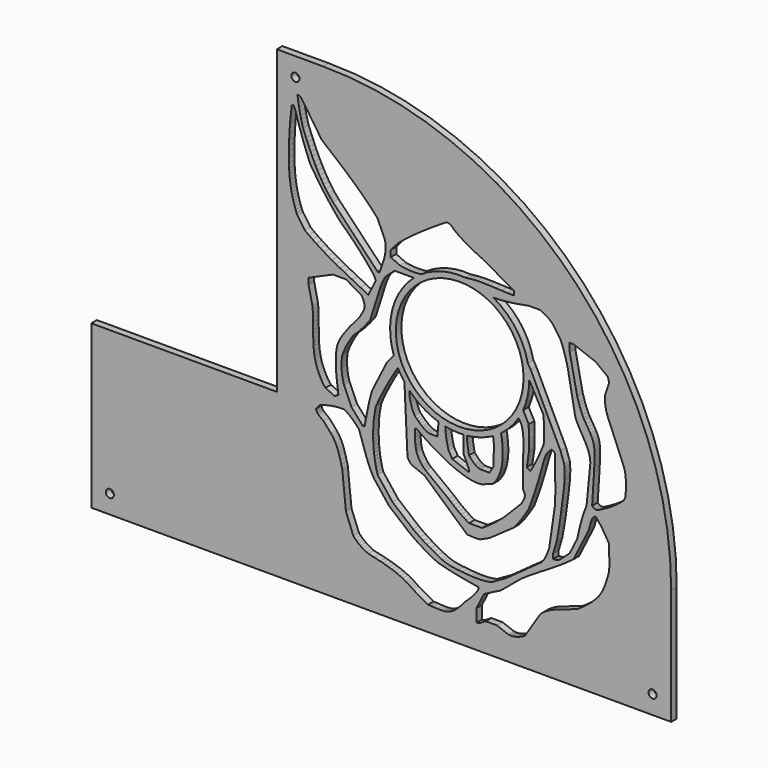
from build123d import *

# Parameters (mm, degrees)
F0_R     = 1.75
F0_R_2   = 27.531271
F1_DEPTH = 3


# Not quite as in the source:
# - ends of sketch curves that miss each other by under 0.0002 mm in the source are joined


with BuildPart() as f1:
    # F0 (on Front) → F1 (new body)
    with BuildSketch(Plane.XZ):
        with BuildLine():
            Line((-25, 100), (-45, 100))
            Line((-45, 100), (-45, -30))
            Line((-45, -30), (-125, -30))
            Line((-125, -30), (-125, -100))
            Line((-125, -100), (125, -100))
            Line((125, -100), (125, -50))
            ThreePointArc((125, -50), (81.066017178, 56.066017178), (-25, 100))
        make_face()
        with Locations((-117, -92)):
            Circle(F0_R, mode=Mode.SUBTRACT)
        Polygon((-31.287949, 17.776814), (-20.835395, 22.366186), (-15.207096, 22.366186), (-8.774755, 18.694689), (-8.557255, 18.433574), (-8.358189, 18.168406), (-8.176948, 17.89932), (-8.012925, 17.626449), (-7.865514, 17.349925), (-7.734107, 17.069883), (-7.618096, 16.786456), (-7.516876, 16.499777), (-7.356374, 15.9172), (-7.247744, 15.323219), (-7.186129, 14.718902), (-7.16667, 14.105317), (-7.502032, 13.354527), (-7.849095, 12.614687), (-8.211531, 11.889235), (-8.593012, 11.181607), (-8.997212, 10.495239), (-9.427801, 9.833569), (-9.888453, 9.200034), (-10.38284, 8.59807), (-13.599011, 4.926573), (-14.451265, 3.745074), (-15.324612, 2.564526), (-16.187258, 1.372942), (-16.604634, 0.769266), (-17.007414, 0.158336), (-17.391623, -0.461346), (-17.753288, -1.091279), (-18.088435, -1.732961), (-18.39309, -2.38789), (-18.663278, -3.057565), (-18.895027, -3.743484), (-19.084362, -4.447144), (-19.227309, -5.170046), (-19.379026, -6.24827), (-19.488623, -7.330374), (-19.559357, -8.415861), (-19.594481, -9.504236), (-19.597251, -10.595003), (-19.570922, -11.687668), (-19.518749, -12.781734), (-19.443987, -13.876707), (-19.34989, -14.97209), (-19.239714, -16.067389), (-18.984143, -18.255751), (-18.423267, -22.609659), (-20.031352, -23.527533), (-24.051565, -21.691785), (-24.559491, -21.073539), (-25.027916, -20.429124), (-25.461461, -19.761602), (-25.864748, -19.074035), (-26.242397, -18.369483), (-26.599031, -17.651009), (-26.93927, -16.921673), (-27.267736, -16.184538), (-27.549789, -15.504402), (-27.80476, -14.816116), (-28.034023, -14.120071), (-28.238954, -13.416661), (-28.420928, -12.706275), (-28.581319, -11.989306), (-28.721501, -11.266144), (-28.842851, -10.537182), (-28.946742, -9.802812), (-29.03455, -9.063423), (-29.167415, -7.571159), (-29.252444, -6.063523), (-29.300635, -4.543646), (-29.322988, -3.014661), (-29.330501, -1.479699), (-29.345002, 1.595628), (-29.373987, 3.129728), (-29.432126, 4.657278), (-29.530419, 6.175144), (-29.679864, 7.680196), (-31.287949, 15.023191), align=None, mode=Mode.SUBTRACT)
        Polygon((-17.33139, -27.224259), (-16.011139, -27.199031), (-15.552943, -27.469295), (-15.103782, -27.751451), (-14.231239, -28.349693), (-13.390862, -28.990273), (-12.580003, -29.669707), (-11.796014, -30.384509), (-11.036249, -31.131194), (-10.298059, -31.906279), (-9.578798, -32.706277), (-8.856422, -34.825598), (-8.152829, -36.957361), (-7.44696, -39.087617), (-6.717758, -41.202414), (-6.337826, -42.249657), (-5.944164, -43.287804), (-5.53414, -44.315111), (-5.105121, -45.329834), (-4.654476, -46.33023), (-4.179572, -47.314555), (-3.677776, -48.281065), (-3.146457, -49.228017), (3.285885, -57.488886), (12.130354, -64.831881), (13.575378, -65.896058), (15.042077, -66.909543), (16.528551, -67.876781), (18.032897, -68.802218), (19.553215, -69.6903), (21.087605, -70.545473), (22.634164, -71.372184), (24.190993, -72.174876), (26.382616, -72.770954), (28.581654, -73.31486), (30.787186, -73.813088), (32.998288, -74.272132), (35.214037, -74.698489), (37.433509, -75.098651), (39.655782, -75.479115), (41.879931, -75.846374), (41.879931, -76.764248), (41.589377, -77.243893), (41.287323, -77.708872), (40.974487, -78.160098), (40.651581, -78.598481), (39.978425, -79.440371), (39.273575, -80.241836), (38.542751, -81.010173), (37.791672, -81.752678), (37.02606, -82.476644), (36.251633, -83.189369), (35.355307, -84.217706), (34.44471, -85.245054), (33.511446, -86.239737), (33.033689, -86.714929), (32.547117, -87.170077), (32.050679, -87.60122), (31.543326, -88.004399), (31.024008, -88.375654), (30.491675, -88.711026), (29.945278, -89.006555), (29.383768, -89.258282), (28.806094, -89.462247), (28.211206, -89.61449), (27.715774, -89.704496), (27.218513, -89.771301), (26.719612, -89.817304), (26.219261, -89.844906), (25.214965, -89.854507), (24.207137, -89.819304), (22.18694, -89.691295), (21.177599, -89.636892), (20.17078, -89.61449), (13.738439, -85.942992), (13.194491, -85.539999), (12.644397, -85.153792), (12.088389, -84.783813), (11.526702, -84.429503), (10.959569, -84.090301), (10.387223, -83.76565), (9.227827, -83.15776), (8.050382, -82.601361), (6.856755, -82.09198), (5.648815, -81.625142), (4.428429, -81.196375), (3.197465, -80.801206), (1.95779, -80.435161), (0.711273, -80.093766), (-0.54022, -79.77255), (-3.050659, -79.172757), (-5.558584, -78.599997), (-6.457527, -78.203947), (-7.335221, -77.75418), (-8.188733, -77.252179), (-9.015132, -76.699429), (-9.811483, -76.097415), (-10.574854, -75.44762), (-11.302313, -74.751528), (-11.990926, -74.010625), (-15.207096, -65.749756), (-16.815181, -50.145891), (-17.222247, -48.5181), (-17.644987, -46.891312), (-18.103559, -45.284488), (-18.352581, -44.494488), (-18.618121, -43.716591), (-18.902698, -42.953166), (-19.208831, -42.206583), (-19.539042, -41.479214), (-19.895849, -40.773428), (-20.281772, -40.091596), (-20.699331, -39.436087), (-21.151046, -38.809273), (-21.639437, -38.213524), (-24.855608, -34.542026), (-25.389784, -34.150193), (-25.939985, -33.756238), (-26.479319, -33.351638), (-26.980894, -32.927865), (-27.209118, -32.706124), (-27.417819, -32.476393), (-27.603634, -32.237606), (-27.763202, -31.988697), (-27.893162, -31.728601), (-27.990152, -31.456251), (-28.050812, -31.170582), (-28.071778, -30.870529), (-26.463693, -29.03478), (-25.818544, -28.7986), (-25.172194, -28.58034), (-24.524669, -28.379631), (-23.875993, -28.196101), (-23.226191, -28.029381), (-22.575288, -27.879101), (-21.923308, -27.74489), (-21.270276, -27.626378), (-20.616218, -27.523195), (-19.961157, -27.434971), (-18.648129, -27.301919), align=None, mode=Mode.SUBTRACT)
        with Locations((117, -92)):
            Circle(F0_R, mode=Mode.SUBTRACT)
        Polygon((92.357364, -32.717578), (92.534618, -32.706277), (93.335017, -33.659188), (94.098567, -34.642419), (94.829855, -35.652194), (95.533468, -36.68474), (96.213994, -37.736283), (96.876019, -38.803048), (98.162916, -40.967147), (98.180748, -42.345341), (98.224052, -43.725509), (98.325946, -46.48703), (98.353967, -47.866014), (98.346325, -49.242233), (98.324354, -49.928936), (98.287736, -50.614503), (98.23456, -51.298787), (98.162916, -51.98164), (97.725667, -53.479835), (97.274925, -54.976121), (96.793754, -56.454111), (96.536465, -57.181125), (96.265217, -57.897421), (95.977893, -58.600949), (95.672376, -59.289663), (95.346548, -59.961513), (94.998294, -60.614453), (94.625495, -61.246432), (94.226035, -61.855404), (93.797795, -62.439321), (93.33866, -62.996133), (92.840296, -63.551141), (92.332649, -64.089762), (91.816155, -64.612763), (91.291249, -65.12091), (90.758363, -65.61497), (90.217932, -66.095709), (89.116173, -67.020293), (87.989446, -67.900793), (86.841224, -68.743344), (85.674982, -69.554078), (84.494191, -70.339128), (74.041637, -74.010625), (73.269796, -74.367475), (72.506218, -74.736675), (71.75653, -75.126636), (71.026358, -75.545764), (70.321327, -76.002469), (69.979997, -76.24754), (69.647063, -76.505158), (69.323227, -76.776374), (69.009192, -77.06224), (68.705661, -77.363806), (68.413339, -77.682123), (61.980997, -87.778741), (61.097449, -88.260871), (60.204681, -88.696077), (59.755343, -88.892136), (59.304303, -89.071727), (58.851763, -89.233271), (58.397925, -89.375189), (57.942989, -89.495901), (57.487157, -89.593829), (57.030629, -89.667393), (56.573609, -89.715014), (56.116295, -89.735113), (55.658891, -89.726112), (55.201597, -89.686431), (54.744614, -89.61449), (49.920358, -87.778741), (45.096102, -87.778741), (43.488017, -88.696616), (43.180232, -88.935718), (42.879269, -89.133415), (42.582612, -89.292643), (42.287745, -89.416337), (41.992155, -89.507433), (41.693325, -89.568866), (41.388742, -89.603573), (41.075889, -89.61449), (41.075889, -84.107244), (44.292059, -77.682123), (51.528443, -74.010625), (60.372912, -66.66763), (61.767698, -65.705074), (63.173221, -64.766122), (64.587532, -63.846994), (66.008681, -62.943907), (68.863693, -61.170732), (71.72266, -59.416346), (74.569982, -57.650496), (75.984403, -56.753818), (77.390063, -55.842929), (78.785013, -54.914049), (80.167304, -53.963395), (81.534985, -52.987186), (82.886106, -51.98164), (89.318447, -39.131398), (89.478349, -38.645202), (89.629902, -38.13397), (89.919812, -37.067533), (90.211888, -35.994345), (90.366148, -35.474677), (90.52984, -34.976669), (90.705929, -34.508103), (90.897379, -34.076763), (91.107153, -33.690431), (91.338215, -33.356889), (91.462655, -33.212347), (91.593529, -33.08392), (91.731206, -32.972583), (91.876058, -32.879307), (92.028454, -32.805066), (92.188766, -32.750832), align=None, mode=Mode.SUBTRACT)
        with BuildLine():
            Line((5.863845, -6.032569), (7.17399, -3.901237))
            ThreePointArc((7.17399, -3.901237), (8.4885700791, -6.1926802555), (9.9996377373, -8.359592201))
            Line((9.9996377373, -8.359592201), (11.326311, -36.377775))
            Line((11.326311, -36.377775), (11.549613, -36.847067))
            Line((11.549613, -36.847067), (11.794695, -37.283588))
            Line((11.794695, -37.283588), (12.061841, -37.685854))
            Line((12.061841, -37.685854), (12.351334, -38.052381))
            Line((12.351334, -38.052381), (12.663457, -38.381683))
            Line((12.663457, -38.381683), (12.998494, -38.672276))
            Line((12.998494, -38.672276), (13.356726, -38.922676))
            Line((13.356726, -38.922676), (13.738439, -39.131398))
            Line((13.738439, -39.131398), (18.562695, -40.967147))
            Line((18.562695, -40.967147), (37.055676, -57.488886))
            Line((37.055676, -57.488886), (37.760371, -57.504072))
            Line((37.760371, -57.504072), (38.466722, -57.540951))
            Line((38.466722, -57.540951), (39.880417, -57.627725))
            Line((39.880417, -57.627725), (40.585775, -57.651588))
            Line((40.585775, -57.651588), (41.288815, -57.645079))
            Line((41.288815, -57.645079), (41.988546, -57.595184))
            Line((41.988546, -57.595184), (42.33686, -57.549899))
            Line((42.33686, -57.549899), (42.683974, -57.488886))
            Line((42.683974, -57.488886), (46.704187, -55.653137))
            Line((46.704187, -55.653137), (57.156742, -48.310142))
            Line((57.156742, -48.310142), (58.059534, -47.24523))
            Line((58.059534, -47.24523), (58.929234, -46.152693))
            Line((58.929234, -46.152693), (59.76828, -45.034569))
            Line((59.76828, -45.034569), (60.579112, -43.892893))
            Line((60.579112, -43.892893), (61.364169, -42.729702))
            Line((61.364169, -42.729702), (62.12589, -41.547032))
            Line((62.12589, -41.547032), (62.866715, -40.346918))
            Line((62.866715, -40.346918), (63.589083, -39.131398))
            Line((63.589083, -39.131398), (64.52444, -36.657526))
            Line((64.52444, -36.657526), (65.414147, -34.166174))
            Line((65.414147, -34.166174), (66.26227, -31.658899))
            Line((66.26227, -31.658899), (67.072875, -29.137257))
            Line((67.072875, -29.137257), (67.850027, -26.602805))
            Line((67.850027, -26.602805), (68.597791, -24.057101))
            Line((68.597791, -24.057101), (69.320235, -21.501701))
            Line((69.320235, -21.501701), (70.021424, -18.938162))
            Line((70.021424, -18.938162), (70.354802, -17.949607))
            Line((70.354802, -17.949607), (70.686573, -16.975509))
            Line((70.686573, -16.975509), (70.874061, -16.509192))
            Line((70.874061, -16.509192), (71.087792, -16.064863))
            Line((71.087792, -16.064863), (71.336647, -15.648645))
            Line((71.336647, -15.648645), (71.477022, -15.452992))
            Line((71.477022, -15.452992), (71.629509, -15.266664))
            Line((71.629509, -15.266664), (73.237594, -13.430915))
            Line((73.237594, -13.430915), (73.498671, -13.450513))
            Line((73.498671, -13.450513), (73.736898, -13.506304))
            Line((73.736898, -13.506304), (73.955117, -13.593782))
            Line((73.955117, -13.593782), (74.156175, -13.708441))
            Line((74.156175, -13.708441), (74.342916, -13.845777))
            Line((74.342916, -13.845777), (74.518183, -14.001284))
            Line((74.518183, -14.001284), (74.84568, -14.34879))
            Line((74.84568, -14.34879), (74.864761, -16.873805))
            Line((74.864761, -16.873805), (74.9111, -19.400049))
            Line((74.9111, -19.400049), (75.020133, -24.453277))
            Line((75.020133, -24.453277), (75.050117, -26.978784))
            Line((75.050117, -26.978784), (75.04194, -29.502569))
            Line((75.04194, -29.502569), (75.018429, -30.763586))
            Line((75.018429, -30.763586), (74.979245, -32.023896))
            Line((74.979245, -32.023896), (74.922344, -33.283407))
            Line((74.922344, -33.283407), (74.84568, -34.542026))
            Line((74.84568, -34.542026), (72.433552, -51.063765))
            Line((72.433552, -51.063765), (72.120958, -51.94488))
            Line((72.120958, -51.94488), (71.797544, -52.81656))
            Line((71.797544, -52.81656), (71.455945, -53.672384))
            Line((71.455945, -53.672384), (71.088796, -54.50593))
            Line((71.088796, -54.50593), (70.68873, -55.310776))
            Line((70.68873, -55.310776), (70.248383, -56.080498))
            Line((70.248383, -56.080498), (70.010802, -56.450181))
            Line((70.010802, -56.450181), (69.760388, -56.808676))
            Line((69.760388, -56.808676), (69.496222, -57.155178))
            Line((69.496222, -57.155178), (69.217381, -57.488886))
            Line((69.217381, -57.488886), (53.940571, -68.503379))
            Line((53.940571, -68.503379), (47.50823, -72.174876))
            Line((47.50823, -72.174876), (46.617589, -72.350746))
            Line((46.617589, -72.350746), (45.722921, -72.49229))
            Line((45.722921, -72.49229), (44.824692, -72.601839))
            Line((44.824692, -72.601839), (43.923368, -72.681724))
            Line((43.923368, -72.681724), (43.019414, -72.734276))
            Line((43.019414, -72.734276), (42.113295, -72.761824))
            Line((42.113295, -72.761824), (41.205477, -72.7667))
            Line((41.205477, -72.7667), (40.296425, -72.751235))
            Line((40.296425, -72.751235), (39.386606, -72.717758))
            Line((39.386606, -72.717758), (38.476484, -72.668601))
            Line((38.476484, -72.668601), (36.657193, -72.532567))
            Line((36.657193, -72.532567), (34.842278, -72.361777))
            Line((34.842278, -72.361777), (33.035462, -72.174876))
            Line((33.035462, -72.174876), (32.109897, -72.066438))
            Line((32.109897, -72.066438), (31.185417, -71.932108))
            Line((31.185417, -71.932108), (30.264482, -71.767542))
            Line((30.264482, -71.767542), (29.349552, -71.568395))
            Line((29.349552, -71.568395), (28.443086, -71.330324))
            Line((28.443086, -71.330324), (27.547545, -71.048985))
            Line((27.547545, -71.048985), (26.665389, -70.720034))
            Line((26.665389, -70.720034), (25.799079, -70.339128))
            Line((25.799079, -70.339128), (24.233624, -69.531728))
            Line((24.233624, -69.531728), (22.680461, -68.700864))
            Line((22.680461, -68.700864), (21.141712, -67.842486))
            Line((21.141712, -67.842486), (19.619499, -66.952545))
            Line((19.619499, -66.952545), (18.115943, -66.026989))
            Line((18.115943, -66.026989), (16.633166, -65.061769))
            Line((16.633166, -65.061769), (15.173291, -64.052833))
            Line((15.173291, -64.052833), (13.738439, -62.996133))
            Line((13.738439, -62.996133), (4.89397, -55.653137))
            Line((4.89397, -55.653137), (-1.538371, -47.392268))
            Line((-1.538371, -47.392268), (-1.892653, -46.107249))
            Line((-1.892653, -46.107249), (-2.208281, -44.814068))
            Line((-2.208281, -44.814068), (-2.486289, -43.513491))
            Line((-2.486289, -43.513491), (-2.727707, -42.206282))
            Line((-2.727707, -42.206282), (-2.933569, -40.893208))
            Line((-2.933569, -40.893208), (-3.104906, -39.575033))
            Line((-3.104906, -39.575033), (-3.24275, -38.252523))
            Line((-3.24275, -38.252523), (-3.348133, -36.926443))
            Line((-3.348133, -36.926443), (-3.422087, -35.59756))
            Line((-3.422087, -35.59756), (-3.465645, -34.266638))
            Line((-3.465645, -34.266638), (-3.479838, -32.934442))
            Line((-3.479838, -32.934442), (-3.465699, -31.601739))
            Line((-3.465699, -31.601739), (-3.424259, -30.269293))
            Line((-3.424259, -30.269293), (-3.356551, -28.937871))
            Line((-3.356551, -28.937871), (-3.263606, -27.608237))
            Line((-3.263606, -27.608237), (-3.146457, -26.281157))
            Line((-3.146457, -26.281157), (-2.342414, -21.691785))
            Line((-2.342414, -21.691785), (-1.291097, -19.361952))
            Line((-1.291097, -19.361952), (-0.195246, -17.066275))
            Line((-0.195246, -17.066275), (0.942621, -14.802819))
            Line((0.942621, -14.802819), (2.119983, -12.569653))
            Line((2.119983, -12.569653), (3.334321, -10.364845))
            Line((3.334321, -10.364845), (4.583115, -8.186461))
            Line((4.583115, -8.186461), (5.863845, -6.032569))
        make_face(mode=Mode.SUBTRACT)
        with BuildLine():
            Line((51.747927, -14.98657), (51.560959, -14.330854))
            ThreePointArc((51.560959, -14.330854), (55.7585739676, -10.6035671119), (59.1883085003, -6.1595193162))
            Line((59.1883085003, -6.1595193162), (59.503375, -6.582854))
            Line((59.503375, -6.582854), (59.805742, -7.018074))
            Line((59.805742, -7.018074), (60.095543, -7.465054))
            Line((60.095543, -7.465054), (60.372912, -7.923669))
            Line((60.372912, -7.923669), (60.617881, -8.740815))
            Line((60.617881, -8.740815), (60.81852, -9.568315))
            Line((60.81852, -9.568315), (60.978763, -10.405189))
            Line((60.978763, -10.405189), (61.102548, -11.250456))
            Line((61.102548, -11.250456), (61.193811, -12.103138))
            Line((61.193811, -12.103138), (61.256488, -12.962255))
            Line((61.256488, -12.962255), (61.294514, -13.826827))
            Line((61.294514, -13.826827), (61.311826, -14.695874))
            Line((61.311826, -14.695874), (61.300054, -16.443474))
            Line((61.300054, -16.443474), (61.252658, -18.197217))
            Line((61.252658, -18.197217), (61.201129, -19.949267))
            Line((61.201129, -19.949267), (61.176955, -21.691785))
            Line((61.176955, -21.691785), (61.176955, -32.706277))
            Line((61.176955, -32.706277), (61.449476, -33.059339))
            Line((61.449476, -33.059339), (61.654001, -33.414195))
            Line((61.654001, -33.414195), (61.795876, -33.770209))
            Line((61.795876, -33.770209), (61.880452, -34.126742))
            Line((61.880452, -34.126742), (61.913076, -34.483157))
            Line((61.913076, -34.483157), (61.899098, -34.838816))
            Line((61.899098, -34.838816), (61.843867, -35.193081))
            Line((61.843867, -35.193081), (61.75273, -35.545315))
            Line((61.75273, -35.545315), (61.631038, -35.89488))
            Line((61.631038, -35.89488), (61.484138, -36.241137))
            Line((61.484138, -36.241137), (61.317379, -36.58345))
            Line((61.317379, -36.58345), (61.13611, -36.921181))
            Line((61.13611, -36.921181), (60.751438, -37.580344))
            Line((60.751438, -37.580344), (60.372912, -38.213524))
            Line((60.372912, -38.213524), (53.136528, -45.556519))
            Line((53.136528, -45.556519), (51.987119, -46.579041))
            Line((51.987119, -46.579041), (50.81889, -47.566801))
            Line((50.81889, -47.566801), (49.633158, -48.52223))
            Line((49.633158, -48.52223), (48.431238, -49.447759))
            Line((48.431238, -49.447759), (47.214448, -50.34582))
            Line((47.214448, -50.34582), (45.984103, -51.218846))
            Line((45.984103, -51.218846), (44.741521, -52.069266))
            Line((44.741521, -52.069266), (43.488017, -52.899514))
            Line((43.488017, -52.899514), (37.859718, -52.899514))
            Line((37.859718, -52.899514), (36.684364, -52.207807))
            Line((36.684364, -52.207807), (35.528412, -51.485124))
            Line((35.528412, -51.485124), (34.392131, -50.731033))
            Line((34.392131, -50.731033), (33.275792, -49.945105))
            Line((33.275792, -49.945105), (32.179664, -49.126908))
            Line((32.179664, -49.126908), (31.104018, -48.276011))
            Line((31.104018, -48.276011), (30.049123, -47.391983))
            Line((30.049123, -47.391983), (29.015249, -46.474393))
            Line((29.015249, -46.474393), (19.366737, -39.131398))
            Line((19.366737, -39.131398), (19.021855, -38.857092))
            Line((19.021855, -38.857092), (18.69227, -38.571365))
            Line((18.69227, -38.571365), (18.377378, -38.274667))
            Line((18.377378, -38.274667), (18.076577, -37.96745))
            Line((18.076577, -37.96745), (17.789264, -37.650162))
            Line((17.789264, -37.650162), (17.514835, -37.323255))
            Line((17.514835, -37.323255), (17.002218, -36.642382))
            Line((17.002218, -36.642382), (16.533903, -35.928434))
            Line((16.533903, -35.928434), (16.105065, -35.185011))
            Line((16.105065, -35.185011), (15.71088, -34.415717))
            Line((15.71088, -34.415717), (15.346524, -33.624152))
            Line((15.346524, -33.624152), (15.188098, -33.075231))
            Line((15.188098, -33.075231), (15.051694, -32.520593))
            Line((15.051694, -32.520593), (14.935683, -31.960755))
            Line((14.935683, -31.960755), (14.838438, -31.396236))
            Line((14.838438, -31.396236), (14.758329, -30.827553))
            Line((14.758329, -30.827553), (14.693729, -30.255225))
            Line((14.693729, -30.255225), (14.604543, -29.101705))
            Line((14.604543, -29.101705), (14.557851, -27.939819))
            Line((14.557851, -27.939819), (14.540628, -26.773711))
            Line((14.540628, -26.773711), (14.542482, -24.445408))
            Line((14.542482, -24.445408), (15.346524, -24.445408))
            Line((15.346524, -24.445408), (16.253348, -25.122717))
            Line((16.253348, -25.122717), (17.16887, -25.78186))
            Line((17.16887, -25.78186), (18.092597, -26.423769))
            Line((18.092597, -26.423769), (19.024036, -27.049375))
            Line((19.024036, -27.049375), (19.962693, -27.65961))
            Line((19.962693, -27.65961), (20.908077, -28.255405))
            Line((20.908077, -28.255405), (22.817048, -29.407404))
            Line((22.817048, -29.407404), (24.747004, -30.512825))
            Line((24.747004, -30.512825), (26.694001, -31.579121))
            Line((26.694001, -31.579121), (28.654093, -32.613746))
            Line((28.654093, -32.613746), (30.623334, -33.624152))
            Line((30.623334, -33.624152), (32.198398, -34.225198))
            Line((32.198398, -34.225198), (33.78503, -34.813945))
            Line((33.78503, -34.813945), (34.582351, -35.094162))
            Line((34.582351, -35.094162), (35.382164, -35.359851))
            Line((35.382164, -35.359851), (36.184336, -35.607194))
            Line((36.184336, -35.607194), (36.988733, -35.832374))
            Line((36.988733, -35.832374), (37.795223, -36.031571))
            Line((37.795223, -36.031571), (38.60367, -36.20097))
            Line((38.60367, -36.20097), (39.413943, -36.336751))
            Line((39.413943, -36.336751), (40.225908, -36.435097))
            Line((40.225908, -36.435097), (41.039431, -36.492191))
            Line((41.039431, -36.492191), (41.854379, -36.504213))
            Line((41.854379, -36.504213), (42.670619, -36.467347))
            Line((42.670619, -36.467347), (43.488017, -36.377775))
            Line((43.488017, -36.377775), (48.312273, -34.542026))
            Line((48.312273, -34.542026), (48.623297, -34.174022))
            Line((48.623297, -34.174022), (48.920304, -33.796522))
            Line((48.920304, -33.796522), (49.2035, -33.409891))
            Line((49.2035, -33.409891), (49.47309, -33.01449))
            Line((49.47309, -33.01449), (49.72928, -32.610682))
            Line((49.72928, -32.610682), (49.972276, -32.198832))
            Line((49.972276, -32.198832), (50.419506, -31.352451))
            Line((50.419506, -31.352451), (50.816426, -30.478249))
            Line((50.816426, -30.478249), (51.16468, -29.57913))
            Line((51.16468, -29.57913), (51.465913, -28.657995))
            Line((51.465913, -28.657995), (51.72177, -27.717748))
            Line((51.72177, -27.717748), (51.933897, -26.761291))
            Line((51.933897, -26.761291), (52.103937, -25.791527))
            Line((52.103937, -25.791527), (52.233536, -24.811358))
            Line((52.233536, -24.811358), (52.324339, -23.823687))
            Line((52.324339, -23.823687), (52.37799, -22.831417))
            Line((52.37799, -22.831417), (52.396135, -21.83745))
            Line((52.396135, -21.83745), (52.380419, -20.844689))
            Line((52.380419, -20.844689), (52.332486, -19.856036))
            Line((52.332486, -19.856036), (52.239493, -18.455902))
            Line((52.239493, -18.455902), (52.18185, -17.750284))
            Line((52.18185, -17.750284), (52.109402, -17.046437))
            Line((52.109402, -17.046437), (52.016618, -16.348466))
            Line((52.016618, -16.348466), (51.89797, -15.660475))
            Line((51.89797, -15.660475), (51.747927, -14.98657))
        make_face(mode=Mode.SUBTRACT)
        with BuildLine():
            Line((27.668244, -20.575264), (27.582538, -19.47563))
            ThreePointArc((27.582538, -19.47563), (31.4948088563, -20.0420529161), (35.4475900171, -20.089163316))
            Line((35.4475900171, -20.089163316), (35.44759, -27.199031))
            Line((35.44759, -27.199031), (37.055676, -30.870529))
            Line((37.055676, -30.870529), (37.265125, -31.221887))
            Line((37.265125, -31.221887), (37.438305, -31.565459))
            Line((37.438305, -31.565459), (37.577786, -31.904116))
            Line((37.577786, -31.904116), (37.686139, -32.240728))
            Line((37.686139, -32.240728), (37.765938, -32.578166))
            Line((37.765938, -32.578166), (37.819752, -32.919302))
            Line((37.819752, -32.919302), (37.850155, -33.267007))
            Line((37.850155, -33.267007), (37.859718, -33.624152))
            Line((37.859718, -33.624152), (30.623334, -30.870529))
            Line((30.623334, -30.870529), (29.015249, -28.116905))
            Line((29.015249, -28.116905), (28.727045, -27.061647))
            Line((28.727045, -27.061647), (28.474511, -25.997724))
            Line((28.474511, -25.997724), (28.255401, -24.92591))
            Line((28.255401, -24.92591), (28.067467, -23.846983))
            Line((28.067467, -23.846983), (27.908461, -22.761715))
            Line((27.908461, -22.761715), (27.776136, -21.670884))
            Line((27.776136, -21.670884), (27.668244, -20.575264))
        make_face(mode=Mode.SUBTRACT)
        with BuildLine():
            Line((12.115581, -11.418545), (12.103851, -10.822616))
            ThreePointArc((12.103851, -10.822616), (17.9220025219, -15.5691295954), (24.7365780878, -18.7221977238))
            Line((24.7365780878, -18.7221977238), (24.588172, -20.150834))
            Line((24.588172, -20.150834), (24.454007, -21.582476))
            Line((24.454007, -21.582476), (24.190993, -24.445408))
            Line((24.190993, -24.445408), (20.974823, -24.445408))
            Line((20.974823, -24.445408), (20.500148, -24.333292))
            Line((20.500148, -24.333292), (20.040712, -24.18232))
            Line((20.040712, -24.18232), (19.595326, -23.995827))
            Line((19.595326, -23.995827), (19.1628, -23.777147))
            Line((19.1628, -23.777147), (18.741943, -23.529615))
            Line((18.741943, -23.529615), (18.331568, -23.256563))
            Line((18.331568, -23.256563), (17.930482, -22.961327))
            Line((17.930482, -22.961327), (17.537498, -22.647241))
            Line((17.537498, -22.647241), (16.771072, -21.975854))
            Line((16.771072, -21.975854), (16.022773, -21.269075))
            Line((16.022773, -21.269075), (15.283082, -20.553578))
            Line((15.283082, -20.553578), (14.542482, -19.856036))
            Line((14.542482, -19.856036), (14.253309, -19.341068))
            Line((14.253309, -19.341068), (13.981847, -18.817046))
            Line((13.981847, -18.817046), (13.728209, -18.284493))
            Line((13.728209, -18.284493), (13.492505, -17.743931))
            Line((13.492505, -17.743931), (13.27485, -17.195883))
            Line((13.27485, -17.195883), (13.075353, -16.640871))
            Line((13.075353, -16.640871), (12.894129, -16.079417))
            Line((12.894129, -16.079417), (12.731288, -15.512042))
            Line((12.731288, -15.512042), (12.586944, -14.939271))
            Line((12.586944, -14.939271), (12.461208, -14.361624))
            Line((12.461208, -14.361624), (12.354193, -13.779625))
            Line((12.354193, -13.779625), (12.26601, -13.193795))
            Line((12.26601, -13.193795), (12.196772, -12.604657))
            Line((12.196772, -12.604657), (12.146592, -12.012733))
            Line((12.146592, -12.012733), (12.115581, -11.418545))
        make_face(mode=Mode.SUBTRACT)
        with BuildLine():
            Line((37.022116, -20.388913), (37.043372, -19.960102))
            ThreePointArc((37.043372, -19.960102), (42.7590735062, -18.7726604379), (48.1365902944, -16.5007505424))
            Line((48.1365902944, -16.5007505424), (48.312273, -17.102413))
            Line((48.312273, -17.102413), (48.408404, -17.780783))
            Line((48.408404, -17.780783), (48.479754, -18.46174))
            Line((48.479754, -18.46174), (48.528888, -19.145017))
            Line((48.528888, -19.145017), (48.558368, -19.830345))
            Line((48.558368, -19.830345), (48.570759, -20.517458))
            Line((48.570759, -20.517458), (48.568622, -21.206086))
            Line((48.568622, -21.206086), (48.531024, -22.586823))
            Line((48.531024, -22.586823), (48.394304, -25.354719))
            Line((48.394304, -25.354719), (48.336199, -26.737596))
            Line((48.336199, -26.737596), (48.312273, -28.116905))
            Line((48.312273, -28.116905), (46.704187, -30.870529))
            Line((46.704187, -30.870529), (42.683974, -30.870529))
            Line((42.683974, -30.870529), (42.316257, -30.782884))
            Line((42.316257, -30.782884), (41.960693, -30.666459))
            Line((41.960693, -30.666459), (41.61657, -30.523369))
            Line((41.61657, -30.523369), (41.283176, -30.355729))
            Line((41.283176, -30.355729), (40.959796, -30.165654))
            Line((40.959796, -30.165654), (40.645719, -29.955259))
            Line((40.645719, -29.955259), (40.340231, -29.72666))
            Line((40.340231, -29.72666), (40.042619, -29.48197))
            Line((40.042619, -29.48197), (39.468172, -28.952783))
            Line((39.468172, -28.952783), (38.916675, -28.384617))
            Line((38.916675, -28.384617), (38.382425, -27.794393))
            Line((38.382425, -27.794393), (37.859718, -27.199031))
            Line((37.859718, -27.199031), (37.540454, -25.418422))
            Line((37.540454, -25.418422), (37.383228, -24.497038))
            Line((37.383228, -24.497038), (37.24168, -23.567627))
            Line((37.24168, -23.567627), (37.126365, -22.639709))
            Line((37.126365, -22.639709), (37.047838, -21.722802))
            Line((37.047838, -21.722802), (37.016655, -20.826427))
            Line((37.016655, -20.826427), (37.022116, -20.388913))
        make_face(mode=Mode.SUBTRACT)
        with BuildLine():
            Line((63.589083, -7.005794), (61.1882583075, -2.4379279413))
            ThreePointArc((61.1882583075, -2.4379279413), (63.1664348181, 3.6018566404), (63.8278942138, 9.9228260004))
            Line((63.8278942138, 9.9228260004), (70.021424, -1.498548))
            Line((70.021424, -1.498548), (70.04535, -2.877857))
            Line((70.04535, -2.877857), (70.103456, -4.260735))
            Line((70.103456, -4.260735), (70.240176, -7.028631))
            Line((70.240176, -7.028631), (70.277774, -8.409367))
            Line((70.277774, -8.409367), (70.27991, -9.097996))
            Line((70.27991, -9.097996), (70.26752, -9.785108))
            Line((70.26752, -9.785108), (70.238039, -10.470437))
            Line((70.238039, -10.470437), (70.188906, -11.153713))
            Line((70.188906, -11.153713), (70.117555, -11.83467))
            Line((70.117555, -11.83467), (70.021424, -12.513041))
            Line((70.021424, -12.513041), (69.418389, -14.073511))
            Line((69.418389, -14.073511), (68.787656, -15.614987))
            Line((68.787656, -15.614987), (68.128716, -17.137118))
            Line((68.128716, -17.137118), (67.441062, -18.639557))
            Line((67.441062, -18.639557), (66.724185, -20.121954))
            Line((66.724185, -20.121954), (65.977575, -21.58396))
            Line((65.977575, -21.58396), (65.200725, -23.025228))
            Line((65.200725, -23.025228), (64.393125, -24.445408))
            Line((64.393125, -24.445408), (64.132048, -24.42581))
            Line((64.132048, -24.42581), (63.893822, -24.370019))
            Line((63.893822, -24.370019), (63.675603, -24.282541))
            Line((63.675603, -24.282541), (63.474545, -24.167882))
            Line((63.474545, -24.167882), (63.287804, -24.030546))
            Line((63.287804, -24.030546), (63.112536, -23.875039))
            Line((63.112536, -23.875039), (62.78504, -23.527533))
            Line((62.78504, -23.527533), (63.589083, -18.020287))
            Line((63.589083, -18.020287), (63.645765, -17.335351))
            Line((63.645765, -17.335351), (63.687836, -16.649521))
            Line((63.687836, -16.649521), (63.73419, -15.275547))
            Line((63.73419, -15.275547), (63.740236, -13.899106))
            Line((63.740236, -13.899106), (63.718067, -12.520937))
            Line((63.718067, -12.520937), (63.637452, -9.762379))
            Line((63.637452, -9.762379), (63.60319, -8.38347))
            Line((63.60319, -8.38347), (63.589083, -7.005794))
        make_face(mode=Mode.SUBTRACT)
        with BuildLine():
            Line((64.393125, 14.105317), (63.206423, 15.942039))
            ThreePointArc((63.206423, 15.942039), (57.9753430213, 27.6688596726), (48.3203920684, 36.134345124))
            Line((48.3203920684, 36.134345124), (49.287123, 36.144553))
            Line((49.287123, 36.144553), (50.251555, 36.17408))
            Line((50.251555, 36.17408), (51.213825, 36.221773))
            Line((51.213825, 36.221773), (52.174071, 36.286478))
            Line((52.174071, 36.286478), (53.13243, 36.367042))
            Line((53.13243, 36.367042), (54.089039, 36.462312))
            Line((54.089039, 36.462312), (55.997556, 36.692353))
            Line((55.997556, 36.692353), (57.900722, 36.967375))
            Line((57.900722, 36.967375), (59.799632, 37.27815))
            Line((59.799632, 37.27815), (61.695387, 37.615452))
            Line((61.695387, 37.615452), (63.589083, 37.970051))
            Line((63.589083, 37.970051), (68.413339, 37.970051))
            Line((68.413339, 37.970051), (69.18518, 37.613202))
            Line((69.18518, 37.613202), (69.948758, 37.244001))
            Line((69.948758, 37.244001), (70.698445, 36.854041))
            Line((70.698445, 36.854041), (71.428618, 36.434912))
            Line((71.428618, 36.434912), (72.133649, 35.978207))
            Line((72.133649, 35.978207), (72.474978, 35.733136))
            Line((72.474978, 35.733136), (72.807913, 35.475518))
            Line((72.807913, 35.475518), (73.131749, 35.204302))
            Line((73.131749, 35.204302), (73.445784, 34.918436))
            Line((73.445784, 34.918436), (73.749314, 34.616871))
            Line((73.749314, 34.616871), (74.041637, 34.298553))
            Line((74.041637, 34.298553), (77.257808, 29.709181))
            Line((77.257808, 29.709181), (77.767775, 28.487059))
            Line((77.767775, 28.487059), (78.23736, 27.249989))
            Line((78.23736, 27.249989), (78.671333, 25.999738))
            Line((78.671333, 25.999738), (79.074464, 24.738071))
            Line((79.074464, 24.738071), (79.451524, 23.466755))
            Line((79.451524, 23.466755), (79.807282, 22.187554))
            Line((79.807282, 22.187554), (80.473978, 19.612563))
            Line((80.473978, 19.612563), (83.690149, 2.17295))
            Line((83.690149, 2.17295), (84.494191, 0.337201))
            Line((84.494191, 0.337201), (84.935232, -0.51392))
            Line((84.935232, -0.51392), (85.398914, -1.360955))
            Line((85.398914, -1.360955), (86.364592, -3.047343))
            Line((86.364592, -3.047343), (87.332009, -4.731111))
            Line((87.332009, -4.731111), (87.797863, -5.574873))
            Line((87.797863, -5.574873), (88.241944, -6.421411))
            Line((88.241944, -6.421411), (88.65685, -7.271869))
            Line((88.65685, -7.271869), (89.035179, -8.127392))
            Line((89.035179, -8.127392), (89.369527, -8.989121))
            Line((89.369527, -8.989121), (89.652494, -9.858203))
            Line((89.652494, -9.858203), (89.772395, -10.295857))
            Line((89.772395, -10.295857), (89.876676, -10.735779))
            Line((89.876676, -10.735779), (89.964409, -11.17811))
            Line((89.964409, -11.17811), (90.034671, -11.622994))
            Line((90.034671, -11.622994), (90.086535, -12.070573))
            Line((90.086535, -12.070573), (90.119076, -12.520991))
            Line((90.119076, -12.520991), (90.13137, -12.974391))
            Line((90.13137, -12.974391), (90.12249, -13.430915))
            Line((90.12249, -13.430915), (88.514405, -29.952654))
            Line((88.514405, -29.952654), (88.16542, -30.775186))
            Line((88.16542, -30.775186), (87.834805, -31.605189))
            Line((87.834805, -31.605189), (87.521415, -32.442149))
            Line((87.521415, -32.442149), (87.224106, -33.285548))
            Line((87.224106, -33.285548), (86.941733, -34.134871))
            Line((86.941733, -34.134871), (86.673153, -34.989602))
            Line((86.673153, -34.989602), (86.172792, -36.713221))
            Line((86.172792, -36.713221), (85.713869, -38.452277))
            Line((85.713869, -38.452277), (85.28723, -40.20264))
            Line((85.28723, -40.20264), (84.883723, -41.960181))
            Line((84.883723, -41.960181), (84.494191, -43.72077))
            Line((84.494191, -43.72077), (81.278021, -50.145891))
            Line((81.278021, -50.145891), (77.257808, -53.817389))
            Line((77.257808, -53.817389), (76.895319, -54.082164))
            Line((76.895319, -54.082164), (76.514505, -54.291912))
            Line((76.514505, -54.291912), (76.118881, -54.452711))
            Line((76.118881, -54.452711), (75.711962, -54.570642))
            Line((75.711962, -54.570642), (75.297263, -54.651783))
            Line((75.297263, -54.651783), (74.878299, -54.702214))
            Line((74.878299, -54.702214), (74.458585, -54.728014))
            Line((74.458585, -54.728014), (74.041637, -54.735263))
            Line((74.041637, -54.735263), (74.041637, -52.899514))
            Line((74.041637, -52.899514), (75.649722, -47.392268))
            Line((75.649722, -47.392268), (76.159656, -44.657118))
            Line((76.159656, -44.657118), (76.629222, -41.915058))
            Line((76.629222, -41.915058), (77.063187, -39.166903))
            Line((77.063187, -39.166903), (77.466321, -36.41347))
            Line((77.466321, -36.41347), (77.843391, -33.655576))
            Line((77.843391, -33.655576), (78.199164, -30.894035))
            Line((78.199164, -30.894035), (78.865893, -25.363282))
            Line((78.865893, -25.363282), (79.013101, -23.296236))
            Line((79.013101, -23.296236), (79.069225, -22.258465))
            Line((79.069225, -22.258465), (79.103391, -21.220371))
            Line((79.103391, -21.220371), (79.107869, -20.183837))
            Line((79.107869, -20.183837), (79.074932, -19.150744))
            Line((79.074932, -19.150744), (78.996849, -18.122976))
            Line((78.996849, -18.122976), (78.865893, -17.102413))
            Line((78.865893, -17.102413), (77.257808, -12.513041))
            Line((77.257808, -12.513041), (64.393125, 14.105317))
        make_face(mode=Mode.SUBTRACT)
        Polygon((81.278021, 26.037684), (81.278021, 29.709181), (82.886106, 29.709181), (92.534618, 26.037684), (97.358874, 22.366186), (97.602783, 22.048549), (97.792137, 21.720806), (97.933728, 21.384214), (98.034346, 21.040032), (98.100782, 20.689518), (98.139829, 20.33393), (98.158276, 19.974525), (98.162916, 19.612563), (96.554831, 15.023191), (96.501598, 14.563687), (96.465575, 14.101975), (96.446032, 13.638543), (96.442237, 13.173883), (96.478966, 12.24283), (96.569913, 11.312733), (96.709227, 10.387506), (96.891059, 9.471064), (97.109558, 8.567322), (97.358874, 7.680196), (104.595257, -9.759418), (104.811077, -10.408201), (104.99008, -11.066113), (105.135424, -11.732328), (105.25027, -12.406023), (105.337776, -13.086374), (105.4011, -13.772557), (105.443402, -14.463749), (105.46784, -15.159124), (105.475759, -16.559134), (105.450129, -17.965996), (105.416219, -19.373118), (105.3993, -20.77391), (104.595257, -22.609659), (103.944814, -23.188307), (103.284992, -23.745808), (102.616285, -24.283275), (101.939184, -24.801817), (101.254182, -25.302547), (100.561773, -25.786575), (99.862449, -26.255011), (99.156702, -26.708968), (97.727914, -27.577885), (96.27935, -28.402213), (94.814951, -29.19084), (93.33866, -29.952654), (92.984461, -29.989852), (92.641763, -29.976823), (92.312342, -29.916975), (91.997974, -29.813718), (91.700434, -29.670462), (91.421497, -29.490614), (91.162938, -29.277583), (90.926533, -29.03478), (91.730575, -16.184538), (91.790683, -14.921198), (91.861542, -13.65411), (91.92919, -12.385328), (91.979665, -11.116908), (91.999004, -9.850903), (91.973244, -8.589367), (91.939088, -7.960917), (91.888422, -7.334354), (91.819499, -6.709937), (91.730575, -6.08792), (91.619078, -5.504881), (91.47584, -4.936349), (91.303671, -4.381122), (91.105377, -3.837998), (90.883769, -3.305775), (90.641652, -2.783252), (90.381836, -2.269225), (90.107129, -1.762494), (89.524273, -0.76611), (88.91555, 0.215515), (88.303425, 1.191996), (87.710362, 2.17295), (87.436557, 2.657024), (87.176325, 3.147107), (86.693266, 4.143836), (86.254555, 5.1602), (85.853563, 6.193265), (85.48366, 7.240094), (85.138217, 8.297753), (84.494191, 10.433819), align=None, mode=Mode.SUBTRACT)
        with BuildLine():
            Line((5.698013, 32.462805), (14.093878, 32.462805))
            ThreePointArc((14.093878, 32.462805), (4.8638792891, 17.6826351366), (5.4059149292, 0.2656179761))
            Line((5.4059149292, 0.2656179761), (3.92787, -1.516096))
            Line((3.92787, -1.516096), (2.481842, -3.334297))
            Line((2.481842, -3.334297), (-3.950499, -16.184538))
            Line((-3.950499, -16.184538), (-4.456381, -17.993626))
            Line((-4.456381, -17.993626), (-4.923642, -19.812628))
            Line((-4.923642, -19.812628), (-5.356754, -21.640395))
            Line((-5.356754, -21.640395), (-5.760191, -23.475781))
            Line((-5.760191, -23.475781), (-6.138428, -25.317635))
            Line((-6.138428, -25.317635), (-6.495938, -27.16481))
            Line((-6.495938, -27.16481), (-7.16667, -30.870529))
            Line((-7.16667, -30.870529), (-7.970712, -30.870529))
            Line((-7.970712, -30.870529), (-12.794968, -25.363282))
            Line((-12.794968, -25.363282), (-16.011139, -18.020287))
            Line((-16.011139, -18.020287), (-16.215551, -17.364863))
            Line((-16.215551, -17.364863), (-16.398524, -16.700509))
            Line((-16.398524, -16.700509), (-16.560247, -16.028196))
            Line((-16.560247, -16.028196), (-16.700912, -15.348895))
            Line((-16.700912, -15.348895), (-16.820705, -14.663579))
            Line((-16.820705, -14.663579), (-16.919818, -13.973217))
            Line((-16.919818, -13.973217), (-16.99844, -13.278782))
            Line((-16.99844, -13.278782), (-17.056759, -12.581244))
            Line((-17.056759, -12.581244), (-17.094967, -11.881575))
            Line((-17.094967, -11.881575), (-17.113251, -11.180746))
            Line((-17.113251, -11.180746), (-17.111801, -10.479727))
            Line((-17.111801, -10.479727), (-17.090808, -9.779491))
            Line((-17.090808, -9.779491), (-17.050459, -9.081009))
            Line((-17.050459, -9.081009), (-16.990946, -8.385251))
            Line((-16.990946, -8.385251), (-16.912457, -7.693189))
            Line((-16.912457, -7.693189), (-16.815181, -7.005794))
            Line((-16.815181, -7.005794), (-16.346686, -5.751661))
            Line((-16.346686, -5.751661), (-15.834482, -4.532223))
            Line((-15.834482, -4.532223), (-15.281203, -3.345387))
            Line((-15.281203, -3.345387), (-14.689486, -2.189063))
            Line((-14.689486, -2.189063), (-14.061964, -1.061159))
            Line((-14.061964, -1.061159), (-13.401274, 0.040417))
            Line((-13.401274, 0.040417), (-12.710049, 1.117756))
            Line((-12.710049, 1.117756), (-11.990926, 2.17295))
            Line((-11.990926, 2.17295), (-10.993133, 3.110285))
            Line((-10.993133, 3.110285), (-10.022226, 4.075091))
            Line((-10.022226, 4.075091), (-9.078083, 5.067243))
            Line((-9.078083, 5.067243), (-8.160582, 6.086617))
            Line((-8.160582, 6.086617), (-7.269599, 7.133086))
            Line((-7.269599, 7.133086), (-6.405014, 8.206526))
            Line((-6.405014, 8.206526), (-5.566702, 9.306812))
            Line((-5.566702, 9.306812), (-4.754542, 10.433819))
            Line((-4.754542, 10.433819), (-1.538371, 20.530438))
            Line((-1.538371, 20.530438), (-1.217455, 21.614002))
            Line((-1.217455, 21.614002), (-0.885016, 22.690327))
            Line((-0.885016, 22.690327), (-0.535228, 23.755752))
            Line((-0.535228, 23.755752), (-0.162267, 24.806619))
            Line((-0.162267, 24.806619), (0.239691, 25.839267))
            Line((0.239691, 25.839267), (0.676472, 26.850037))
            Line((0.676472, 26.850037), (1.1539, 27.835271))
            Line((1.1539, 27.835271), (1.677799, 28.791307))
            Line((1.677799, 28.791307), (5.698013, 32.462805))
        make_face(mode=Mode.SUBTRACT)
        Polygon((-38.524333, 81.110148), (-37.72029, 81.110148), (-36.916247, 79.274399), (-36.2194, 76.92476), (-35.500849, 74.586248), (-34.756133, 72.261148), (-33.980789, 69.95175), (-33.170357, 67.66034), (-32.320373, 65.389205), (-31.426377, 63.140633), (-30.483906, 60.916911), (-28.993693, 58.61344), (-27.474622, 56.340209), (-25.924285, 54.099743), (-24.340269, 51.894568), (-22.720166, 49.72721), (-21.061564, 47.600195), (-20.217073, 46.552606), (-19.362054, 45.516049), (-18.496204, 44.490841), (-17.619224, 43.477297), (-15.68006, 41.67088), (-13.776506, 39.825021), (-11.909337, 37.93886), (-10.07933, 36.011538), (-8.287263, 34.042194), (-6.53391, 32.029969), (-4.820049, 29.974002), (-3.978171, 28.929346), (-3.146457, 27.873433), (-2.342414, 26.037684), (-5.558584, 19.612563), (-9.060713, 21.392778), (-12.569557, 23.163433), (-16.069623, 24.953632), (-17.811523, 25.865156), (-19.545419, 26.79248), (-21.269374, 27.739242), (-22.981451, 28.70908), (-24.679714, 29.705632), (-26.362226, 30.732535), (-28.027051, 31.793429), (-29.672251, 32.89195), (-31.295891, 34.031737), (-32.896034, 35.216428), (-36.112205, 39.8058), (-36.527015, 40.792097), (-36.91197, 41.786974), (-37.268029, 42.790057), (-37.596148, 43.800972), (-37.897286, 44.819344), (-38.172401, 45.8448), (-38.422449, 46.876964), (-38.648389, 47.915464), (-38.851178, 48.959925), (-39.031774, 50.009972), (-39.191135, 51.065232), (-39.330218, 52.12533), (-39.44998, 53.189892), (-39.551381, 54.258545), (-39.635377, 55.330913), (-39.702926, 56.406623), (-39.792513, 58.566572), (-39.827804, 60.735398), (-39.816461, 62.910108), (-39.766144, 65.087709), (-39.684516, 67.265207), (-39.579238, 69.439609), (-39.328375, 73.767152), align=None, mode=Mode.SUBTRACT)
        Polygon((-35.910149, 84.186802), (-36.112205, 85.69952), (-35.858821, 85.688682), (-35.62679, 85.657148), (-35.414469, 85.606383), (-35.220214, 85.537855), (-35.042382, 85.453029), (-34.87933, 85.353372), (-34.729412, 85.240352), (-34.590987, 85.115434), (-34.342039, 84.835772), (-34.119337, 84.526119), (-33.700077, 83.863771), (-25.65965, 71.931404), (-19.385303, 66.727633), (-16.269782, 64.098819), (-14.724322, 62.769116), (-13.189685, 61.425952), (-11.66784, 60.06688), (-10.160755, 58.689454), (-8.670395, 57.291227), (-7.198731, 55.86975), (-5.747728, 54.422579), (-4.319356, 52.947264), (-2.915581, 51.441359), (-1.538371, 49.902418), (1.677799, 42.559423), (1.748119, 42.039866), (1.802173, 41.517508), (1.840003, 40.993042), (1.861649, 40.467161), (1.867151, 39.940559), (1.85655, 39.413927), (1.829886, 38.887961), (1.787199, 38.363352), (1.728531, 37.840795), (1.653921, 37.320982), (1.563411, 36.804606), (1.457039, 36.292362), (1.334848, 35.784941), (1.196877, 35.283037), (1.043166, 34.787343), (0.873757, 34.298553), (-0.734329, 29.709181), (-1.538371, 29.709181), (-20.835395, 49.902418), (-21.381545, 50.538712), (-21.914802, 51.185435), (-22.435524, 51.842249), (-22.944071, 52.508817), (-23.926078, 53.869874), (-24.863699, 55.265914), (-25.759811, 56.694244), (-26.617291, 58.152172), (-27.439014, 59.637007), (-28.227857, 61.146057), (-28.986696, 62.676629), (-29.718408, 64.226032), (-30.425868, 65.791575), (-31.111954, 67.370564), (-31.779542, 68.960308), (-32.431507, 70.558116), (-33.700077, 73.767152), (-34.110425, 75.235532), (-34.487001, 76.7111), (-34.831142, 78.193573), (-35.144189, 79.682664), (-35.42748, 81.17809), (-35.682353, 82.679564), align=None, mode=Mode.SUBTRACT)
        with Locations((-37, 92)):
            Circle(F0_R, mode=Mode.SUBTRACT)
        with Locations((33.827946, 9.867084)):
            Circle(F0_R_2, mode=Mode.SUBTRACT)
        with BuildLine():
            Line((37.575594, 39.935824), (36.290073, 39.765879))
            ThreePointArc((36.290073, 39.765879), (26.3225651975, 38.9130692477), (17.1896432108, 34.8303946838))
            Line((17.1896432108, 34.8303946838), (16.050974, 34.726234))
            Line((16.050974, 34.726234), (14.912468, 34.661161))
            Line((14.912468, 34.661161), (13.774576, 34.637408))
            Line((13.774576, 34.637408), (12.637749, 34.657201))
            Line((12.637749, 34.657201), (11.502441, 34.722771))
            Line((11.502441, 34.722771), (10.369102, 34.836346))
            Line((10.369102, 34.836346), (9.238184, 35.000155))
            Line((9.238184, 35.000155), (8.11014, 35.216428))
            Line((8.11014, 35.216428), (4.089927, 37.052177))
            Line((4.089927, 37.052177), (4.089927, 39.8058))
            Line((4.089927, 39.8058), (7.306098, 43.477297))
            Line((7.306098, 43.477297), (8.5579, 44.504162))
            Line((8.5579, 44.504162), (9.818327, 45.513864))
            Line((9.818327, 45.513864), (11.087094, 46.506968))
            Line((11.087094, 46.506968), (12.363918, 47.484037))
            Line((12.363918, 47.484037), (13.648517, 48.445635))
            Line((13.648517, 48.445635), (14.940607, 49.392325))
            Line((14.940607, 49.392325), (16.239904, 50.324671))
            Line((16.239904, 50.324671), (17.546126, 51.243236))
            Line((17.546126, 51.243236), (20.178211, 53.041279))
            Line((20.178211, 53.041279), (22.834597, 54.790963))
            Line((22.834597, 54.790963), (25.513017, 56.496797))
            Line((25.513017, 56.496797), (28.211206, 58.163288))
            Line((28.211206, 58.163288), (28.478352, 58.153301))
            Line((28.478352, 58.153301), (28.733361, 58.124092))
            Line((28.733361, 58.124092), (28.976944, 58.076786))
            Line((28.976944, 58.076786), (29.209813, 58.01251))
            Line((29.209813, 58.01251), (29.432678, 57.932391))
            Line((29.432678, 57.932391), (29.646252, 57.837554))
            Line((29.646252, 57.837554), (29.851245, 57.729127))
            Line((29.851245, 57.729127), (30.048368, 57.608235))
            Line((30.048368, 57.608235), (30.421849, 57.333563))
            Line((30.421849, 57.333563), (30.772385, 57.022549))
            Line((30.772385, 57.022549), (31.105664, 56.684204))
            Line((31.105664, 56.684204), (31.427377, 56.327539))
            Line((31.427377, 56.327539), (32.188921, 55.760567))
            Line((32.188921, 55.760567), (32.95785, 55.212365))
            Line((32.95785, 55.212365), (33.733794, 54.682))
            Line((33.733794, 54.682), (34.516387, 54.168534))
            Line((34.516387, 54.168534), (35.305259, 53.671032))
            Line((35.305259, 53.671032), (36.100043, 53.188559))
            Line((36.100043, 53.188559), (37.705875, 52.264955))
            Line((37.705875, 52.264955), (39.330937, 51.390237))
            Line((39.330937, 51.390237), (40.972284, 50.556919))
            Line((40.972284, 50.556919), (42.626974, 49.757517))
            Line((42.626974, 49.757517), (44.292059, 48.984544))
            Line((44.292059, 48.984544), (57.156742, 41.641549))
            Line((57.156742, 41.641549), (57.156742, 39.8058))
            Line((57.156742, 39.8058), (55.85281, 39.816651))
            Line((55.85281, 39.816651), (54.54633, 39.84627))
            Line((54.54633, 39.84627), (51.927881, 39.944199))
            Line((51.927881, 39.944199), (49.30571, 40.064363))
            Line((49.30571, 40.064363), (46.684133, 40.171538))
            Line((46.684133, 40.171538), (45.374916, 40.209247))
            Line((45.374916, 40.209247), (44.067465, 40.2305))
            Line((44.067465, 40.2305), (42.762321, 40.230895))
            Line((42.762321, 40.230895), (41.460022, 40.206027))
            Line((41.460022, 40.206027), (40.161109, 40.151495))
            Line((40.161109, 40.151495), (38.866119, 40.062895))
            Line((38.866119, 40.062895), (37.575594, 39.935824))
        make_face(mode=Mode.SUBTRACT)
    extrude(amount=F1_DEPTH)


solid = f1.part
